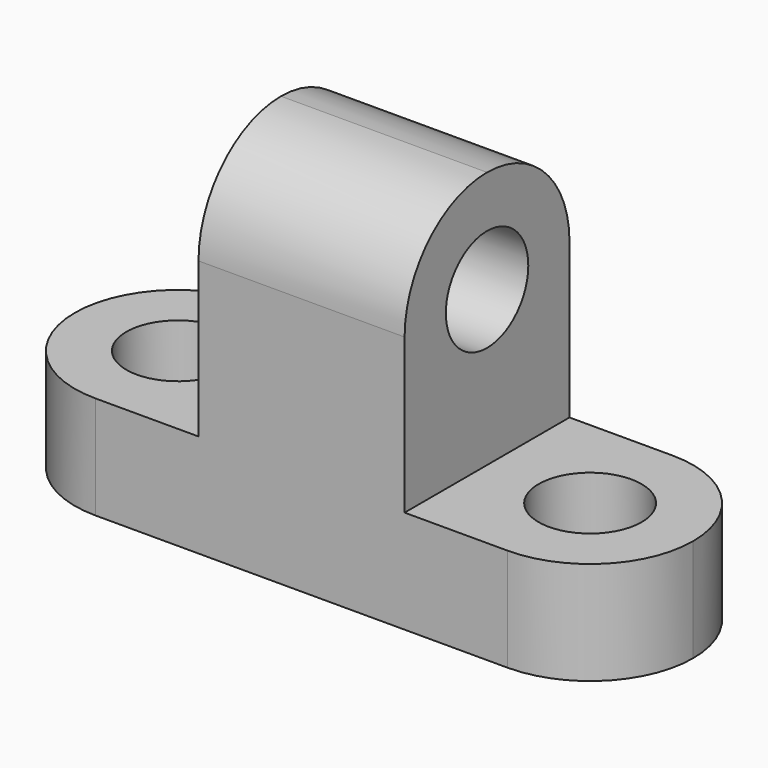
from build123d import *

# Parameters (mm, degrees)
F1_DEPTH  = 25.4
F2_R      = 12.7
F3_R      = 12.69999
F4_R      = 12.7
F5_R      = 12.69999
F6_R      = 12.7
F7_R      = 12.69999
F8_R      = 6.35
F9_DEPTH  = 25.4
F10_R     = 6.35
F11_DEPTH = 25.4
F12_R     = 6.35
F13_DEPTH = 25.4


# Not quite as in the source:
# - a fillet or chamfer is up to 0.001 mm smaller than in the source, because OpenCascade refuses the exact size


with BuildPart() as f1:
    # F0 (on Front) → F1 (new body)
    with BuildSketch(Plane.XZ):
        Polygon((-34.4568602741, 12.7), (-34.4568602741, 0), (41.7431397259, 0), (41.7431397259, 12.7), (16.3431397259, 12.7), (16.3431397259, 44.45), (-9.0568602741, 44.45), (-9.0568602741, 12.7), align=None)
    extrude(amount=F1_DEPTH)

    # F2
    f2_edges = [f1.edges().sort_by_distance(p)[0] for p in [
        (41.74314, -25.4, 6.35),
    ]]
    fillet(f2_edges, radius=F2_R)

    # F3 (radius 12.7 in the source; OpenCascade refuses exactly that, so slightly less here)
    f3_edges = [f1.edges().sort_by_distance(p)[0] for p in [
        (41.74314, 0, 6.35),
    ]]
    fillet(f3_edges, radius=F3_R)

    # F4
    f4_edges = [f1.edges().sort_by_distance(p)[0] for p in [
        (-34.45686, -25.4, 6.35),
    ]]
    fillet(f4_edges, radius=F4_R)

    # F5 (radius 12.7 in the source; OpenCascade refuses exactly that, so slightly less here)
    f5_edges = [f1.edges().sort_by_distance(p)[0] for p in [
        (-34.45686, 0, 6.35),
    ]]
    fillet(f5_edges, radius=F5_R)

    # F6
    f6_edges = [f1.edges().sort_by_distance(p)[0] for p in [
        (3.64314, -25.4, 44.45),
    ]]
    fillet(f6_edges, radius=F6_R)

    # F7 (radius 12.7 in the source; OpenCascade refuses exactly that, so slightly less here)
    f7_edges = [f1.edges().sort_by_distance(p)[0] for p in [
        (3.64314, 0, 44.45),
    ]]
    fillet(f7_edges, radius=F7_R)

    # F8 (on face) → F9 (cut)
    with BuildSketch(Plane.XY.offset(12.7)):
        with Locations((29.0431397259, -12.7)):
            Circle(F8_R)
    extrude(amount=-F9_DEPTH, mode=Mode.SUBTRACT)

    # F10 (on face) → F11 (cut)
    with BuildSketch(Plane.XY.offset(12.7)):
        with Locations((-21.7568602741, -12.7)):
            Circle(F10_R)
    extrude(amount=-F11_DEPTH, mode=Mode.SUBTRACT)

    # F12 (on face) → F13 (cut)
    with BuildSketch(Plane.YZ.offset(16.3431397259)):
        with Locations((-12.7, 31.75)):
            Circle(F12_R)
    extrude(amount=-F13_DEPTH, mode=Mode.SUBTRACT)


solid = f1.part
